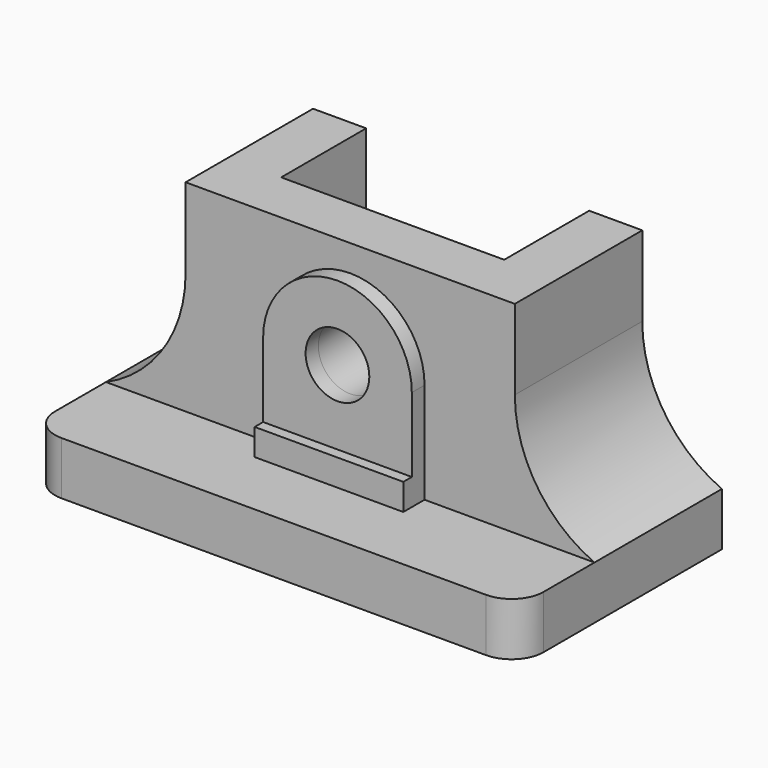
from build123d import *

# Parameters (mm, degrees)
F1_DEPTH    = 48
F2_DEPTH    = 10
F3_R        = 6
F4_T1_DEPTH = 30
F5_T1_DEPTH = 30
F7_DEPTH    = 5
F6_R        = 6
F8_DEPTH    = 3
F9_DEPTH    = 25


# Not quite as in the source:
# - a fillet or chamfer that OpenCascade refuses, or shapes differently, is made with other operations: its cross-section is extruded or revolved along the edge and cut away or added


with BuildPart() as f1:
    # F0 (on Top) → F1 (new body)
    with BuildSketch(Plane.XY):
        Polygon((21, -1.625), (0, -1.625), (-21, -1.625), (-21, 18.375), (-31, 18.375), (-31, -11.625), (0, -11.625), (31, -11.625), (31, 18.375), (21, 18.375), align=None)
    extrude(amount=F1_DEPTH)

    # F0 (on Top) → F2 (join)
    with BuildSketch(Plane.XY):
        Polygon((21, -1.625), (0, -1.625), (-21, -1.625), (-21, 18.375), (-31, 18.375), (-31, -11.625), (0, -11.625), (31, -11.625), (31, 18.375), (21, 18.375), align=None)
        Polygon((-31, -11.625), (-31, 18.375), (-46, 18.375), (-46, -29.625), (0, -29.625), (46, -29.625), (46, 18.375), (31, 18.375), (31, -11.625), (0, -11.625), align=None)
    extrude(amount=F2_DEPTH)

    # F3
    f3_edges = [f1.edges().sort_by_distance(p)[0] for p in [
        (-46, -29.625, 5),
        (46, -29.625, 5),
    ]]
    fillet(f3_edges, radius=F3_R)

    # F4: fillet of radius 25 on 1 edges, made by hand

    # F4_s2 → F4_t1 (join)
    with BuildSketch(Plane.XZ.offset(-18.375)):
        with BuildLine():
            ThreePointArc((46, 10), (35.0834993366, 19.2198145372), (31, 32.9128784748))
            Line((31, 32.9128784748), (31, 10))
            Line((31, 10), (46, 10))
        make_face()
    extrude(amount=F4_T1_DEPTH)

    # F5: fillet of radius 25 on 1 edges, made by hand

    # F5_s2 → F5_t1 (join)
    with BuildSketch(Plane.XZ.offset(-18.375)):
        with BuildLine():
            ThreePointArc((-46, 10), (-35.0834993366, 19.2198145372), (-31, 32.9128784748))
            Line((-31, 32.9128784748), (-31, 10))
            Line((-31, 10), (-46, 10))
        make_face()
    extrude(amount=F5_T1_DEPTH)

    # F6 (on face) → F7 (join)
    with BuildSketch(Plane.XZ.offset(11.625)):
        Polygon((-14, 15), (-14, 10), (14, 10), (14, 15), (0, 15), align=None)
    extrude(amount=F7_DEPTH)

    # F6 (on face) → F8 (join)
    with BuildSketch(Plane.XZ.offset(11.625)):
        Polygon((-14, 15), (-14, 10), (14, 10), (14, 15), (0, 15), align=None)
        with BuildLine():
            Line((-14, 29), (-14, 15))
            Line((-14, 15), (0, 15))
            Line((0, 15), (14, 15))
            Line((14, 15), (14, 29))
            ThreePointArc((14, 29), (0, 43), (-14, 29))
        make_face()
        with Locations((0, 29)):
            Circle(F6_R, mode=Mode.SUBTRACT)
    extrude(amount=F8_DEPTH)

    # F9 (cut): a face of the model
    f9_faces = [f1.faces().sort_by_distance(p)[0] for p in [
        (0, -11.625, 29),
    ]]
    extrude(f9_faces, amount=-F9_DEPTH, mode=Mode.SUBTRACT)


solid = f1.part
